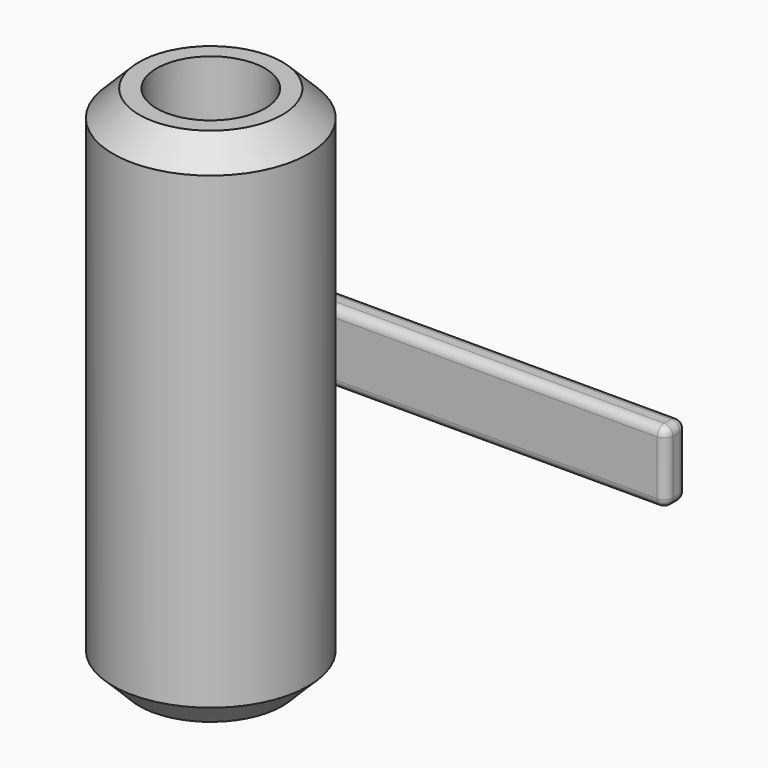
from build123d import *

# Parameters (mm, degrees)
F0_R          = 7.9375
F0_R_2        = 6.35
F2_DEPTH      = 50.8
F3_R          = 14.2875
F3_R_2        = 7.9375
F4_DEPTH      = 63.5
F4_DEPTH_BACK = 12.7
F5_SIZE       = 3.81
F7_START      = -13.97
F6_W          = 64.1522035003
F6_H          = 10.4847997427
F7_DEPTH      = 3.81
F8_T1_DEPTH   = 66.0572035003
F8_T3_DEPTH   = 16.8347997427
F8_T5_DEPTH   = 7.9447997427
F8_T7_DEPTH   = 1.27
F8_S11_W      = 1.27
F8_S11_H      = 1.27
F8_T12_DEPTH  = 1.27
F8_S17_W      = 1.27
F8_S17_H      = 1.27
F8_T18_DEPTH  = 1.27
F8_S23_W      = 1.27
F8_S23_H      = 1.27
F8_T24_DEPTH  = 1.27
F8_S29_W      = 1.27
F8_S29_H      = 1.27
F8_T30_DEPTH  = 1.27
F8_T36_DEPTH  = 54.3607688419
F8_S37_R      = 14.2875
F8_T38_DEPTH  = 29
F8_T42_DEPTH  = 54.3607688419
F8_S43_R      = 14.2875
F8_T44_DEPTH  = 29
F8_T48_DEPTH  = 12.0558566395
F8_S49_R      = 14.2875
F8_T50_DEPTH  = 8
F8_T54_DEPTH  = 12.0558566395
F8_S55_R      = 14.2875
F8_T56_DEPTH  = 8


# Not quite as in the source:
# - a fillet or chamfer that OpenCascade refuses, or shapes differently, is made with other operations: its cross-section is extruded or revolved along the edge and cut away or added
# - a feature names something its author has since deleted; it is built from what else it names


with BuildPart() as f2:
    # F0 (on Top) → F2 (new body)
    with BuildSketch(Plane.XY):
        Circle(F0_R)
        Circle(F0_R_2, mode=Mode.SUBTRACT)
    extrude(amount=F2_DEPTH)

    # F3 (on face) → F4 (join, two sides)
    with BuildSketch(Plane.XY) as f4_sk:
        Circle(F3_R)
        Circle(F3_R_2, mode=Mode.SUBTRACT)
    extrude(amount=F4_DEPTH)
    extrude(f4_sk.sketch, amount=-F4_DEPTH_BACK)

    # F5
    f5_edges = [f2.edges().sort_by_distance(p)[0] for p in [
        (-14.2875, 0, 63.5),
        (-14.2875, 0, -12.7),
    ]]
    chamfer(f5_edges, length=F5_SIZE)

    # F6 (on Front) → F7 (join)
    with BuildSketch(Plane.XZ.offset(F7_START)):
        with Locations((23.3749561012, 26.5372619033)):
            Rectangle(F6_W, F6_H)
    extrude(amount=-F7_DEPTH)

    # F8: fillet of radius 1.27 on 11 edges, made by hand

    # F8_s2 → F8_t1 (cut)
    with BuildSketch(Plane.YZ.offset(-11.876145649)):
        with BuildLine():
            ThreePointArc((16.51, 31.7796617746), (17.4080256121, 31.4076873867), (17.78, 30.5096617746))
            Line((17.78, 30.5096617746), (17.78, 31.7796617746))
            Line((17.78, 31.7796617746), (16.51, 31.7796617746))
        make_face()
        with BuildLine():
            ThreePointArc((16.51, 21.2948620319), (17.4080256121, 21.6668364198), (17.78, 22.5648620319))
            Line((17.78, 22.5648620319), (17.78, 21.2948620319))
            Line((17.78, 21.2948620319), (16.51, 21.2948620319))
        make_face()
    extrude(amount=F8_T1_DEPTH, mode=Mode.SUBTRACT)

    # F8_s4 → F8_t3 (cut)
    with BuildSketch(Plane.XY.offset(18.1198620319)):
        with BuildLine():
            ThreePointArc((-7.431145649, 17.78), (-8.3291712611, 17.4080256121), (-8.701145649, 16.51))
            Line((-8.701145649, 16.51), (-8.701145649, 17.78))
            Line((-8.701145649, 17.78), (-7.431145649, 17.78))
        make_face()
    extrude(amount=F8_T3_DEPTH, mode=Mode.SUBTRACT)

    # F8_s6 → F8_t5 (cut)
    with BuildSketch(Plane.XY.offset(22.5648620319)):
        with BuildLine():
            ThreePointArc((54.1810578513, 13.97), (55.0790834634, 14.3419743879), (55.4510578513, 15.24))
            Line((55.4510578513, 15.24), (55.4510578513, 13.97))
            Line((55.4510578513, 13.97), (54.1810578513, 13.97))
        make_face()
        with BuildLine():
            ThreePointArc((55.4510578513, 16.51), (55.0790834634, 17.4080256121), (54.1810578513, 17.78))
            Line((54.1810578513, 17.78), (55.4510578513, 17.78))
            Line((55.4510578513, 17.78), (55.4510578513, 16.51))
        make_face()
    extrude(amount=F8_T5_DEPTH, mode=Mode.SUBTRACT)

    # F8_s8 → F8_t7 (cut)
    with BuildSketch(Plane.XZ.offset(-16.51)):
        with BuildLine():
            ThreePointArc((54.1810578513, 31.7796617746), (55.0790834634, 31.4076873867), (55.4510578513, 30.5096617746))
            Line((55.4510578513, 30.5096617746), (55.4510578513, 31.7796617746))
            Line((55.4510578513, 31.7796617746), (54.1810578513, 31.7796617746))
        make_face()
        with BuildLine():
            ThreePointArc((54.1810578513, 21.2948620319), (55.0790834634, 21.6668364198), (55.4510578513, 22.5648620319))
            Line((55.4510578513, 22.5648620319), (55.4510578513, 21.2948620319))
            Line((55.4510578513, 21.2948620319), (54.1810578513, 21.2948620319))
        make_face()
    extrude(amount=F8_T7_DEPTH, mode=Mode.SUBTRACT)


with BuildPart() as f8_tool10:
    # F8_s11 → F8_t12 (new body)
    with BuildSketch(Plane.XY.offset(30.5096617746)):
        with Locations((54.8160578513, 17.145)):
            Rectangle(F8_S11_W, F8_S11_H)
    extrude(amount=F8_T12_DEPTH)

    # F8_s13 → F8_t14 (revolve, cut)
    with BuildSketch(Plane(origin=(54.1810578513, 16.51, 30.5096617746), x_dir=(-0.7071067812, -0.7071067812, 0), z_dir=(-0.7071067812, 0.7071067812, 0))):
        with BuildLine():
            ThreePointArc((0, -1.27), (1.27, 0), (0, 1.27))
            Line((0, 1.27), (0, -1.27))
        make_face()
    revolve(axis=Axis((54.1810578513, 16.51, 30.5096617746), (0, 0, 1)), mode=Mode.SUBTRACT)


with BuildPart() as f2_1:
    add(f2.part)

    # F8_t9: cut F8_tool10
    add(f8_tool10.part, mode=Mode.SUBTRACT)


with BuildPart() as f8_tool16:
    # F8_s17 → F8_t18 (new body)
    with BuildSketch(Plane.YZ.offset(54.1810578513)):
        with Locations((17.145, 21.9298620319)):
            Rectangle(F8_S17_W, F8_S17_H)
    extrude(amount=F8_T18_DEPTH)

    # F8_s19 → F8_t20 (revolve, cut)
    with BuildSketch(Plane(origin=(54.1810578513, 16.51, 22.5648620319), x_dir=(0, -0.7071067812, 0.7071067812), z_dir=(0, 0.7071067812, 0.7071067812))):
        with BuildLine():
            ThreePointArc((0, -1.27), (1.27, 0), (0, 1.27))
            Line((0, 1.27), (0, -1.27))
        make_face()
    revolve(axis=Axis((54.1810578513, 16.51, 22.5648620319), (1, 0, 0)), mode=Mode.SUBTRACT)


with BuildPart() as f2_2:
    add(f2_1.part)

    # F8_t15: cut F8_tool16
    add(f8_tool16.part, mode=Mode.SUBTRACT)


with BuildPart() as f8_tool22:
    # F8_s23 → F8_t24 (new body)
    with BuildSketch(Plane.YZ.offset(54.1810578513)):
        with Locations((14.605, 21.9298620319)):
            Rectangle(F8_S23_W, F8_S23_H)
    extrude(amount=F8_T24_DEPTH)

    # F8_s25 → F8_t26 (revolve, cut)
    with BuildSketch(Plane(origin=(54.1810578513, 15.24, 22.5648620319), x_dir=(0, 0.7071067812, 0.7071067812), z_dir=(0, 0.7071067812, -0.7071067812))):
        with BuildLine():
            ThreePointArc((0, -1.27), (1.27, 0), (0, 1.27))
            Line((0, 1.27), (0, -1.27))
        make_face()
    revolve(axis=Axis((54.1810578513, 15.24, 22.5648620319), (1, 0, 0)), mode=Mode.SUBTRACT)


with BuildPart() as f2_3:
    add(f2_2.part)

    # F8_t21: cut F8_tool22
    add(f8_tool22.part, mode=Mode.SUBTRACT)


with BuildPart() as f8_tool28:
    # F8_s29 → F8_t30 (new body)
    with BuildSketch(Plane.XY.offset(30.5096617746)):
        with Locations((54.8160578513, 14.605)):
            Rectangle(F8_S29_W, F8_S29_H)
    extrude(amount=F8_T30_DEPTH)

    # F8_s31 → F8_t32 (revolve, cut)
    with BuildSketch(Plane(origin=(54.1810578513, 15.24, 30.5096617746), x_dir=(-0.7071067812, 0.7071067812, 0), z_dir=(0.7071067812, 0.7071067812, 0))):
        with BuildLine():
            ThreePointArc((0, -1.27), (1.27, 0), (0, 1.27))
            Line((0, 1.27), (0, -1.27))
        make_face()
    revolve(axis=Axis((54.1810578513, 15.24, 30.5096617746), (0, 0, 1)), mode=Mode.SUBTRACT)


with BuildPart() as f2_4:
    add(f2_3.part)

    # F8_t27: cut F8_tool28
    add(f8_tool28.part, mode=Mode.SUBTRACT)


with BuildPart() as f8_tool34:
    # F8_s35 → F8_t36 (new body)
    with BuildSketch(Plane.YZ.offset(-0.1797109906)):
        with BuildLine():
            ThreePointArc((13.97, 22.5648620319), (14.3419743879, 21.6668364198), (15.24, 21.2948620319))
            Line((15.24, 21.2948620319), (13.97, 21.2948620319))
            Line((13.97, 21.2948620319), (13.97, 22.5648620319))
        make_face()
    extrude(amount=F8_T36_DEPTH)

    # F8_s37 → F8_t38 (cut, symmetric)
    with BuildSketch(Plane.XY.offset(21.9)):
        Circle(F8_S37_R)
    extrude(amount=F8_T38_DEPTH, both=True, mode=Mode.SUBTRACT)


with BuildPart() as f2_5:
    add(f2_4.part)

    # F8_t33: cut F8_tool34
    add(f8_tool34.part, mode=Mode.SUBTRACT)


with BuildPart() as f8_tool40:
    # F8_s41 → F8_t42 (new body)
    with BuildSketch(Plane.YZ.offset(54.1810578513)):
        with BuildLine():
            ThreePointArc((13.97, 30.5096617746), (14.3419743879, 31.4076873867), (15.24, 31.7796617746))
            Line((15.24, 31.7796617746), (13.97, 31.7796617746))
            Line((13.97, 31.7796617746), (13.97, 30.5096617746))
        make_face()
    extrude(amount=-F8_T42_DEPTH)

    # F8_s43 → F8_t44 (cut, symmetric)
    with BuildSketch(Plane.XY.offset(31.1)):
        Circle(F8_S43_R)
    extrude(amount=F8_T44_DEPTH, both=True, mode=Mode.SUBTRACT)


with BuildPart() as f2_6:
    add(f2_5.part)

    # F8_t39: cut F8_tool40
    add(f8_tool40.part, mode=Mode.SUBTRACT)


with BuildPart() as f8_tool46:
    # F8_s47 → F8_t48 (new body)
    with BuildSketch(Plane.YZ.offset(-11.876145649)):
        with BuildLine():
            ThreePointArc((15.24, 21.2948620319), (14.3419743879, 21.6668364198), (13.97, 22.5648620319))
            Line((13.97, 22.5648620319), (13.97, 21.2948620319))
            Line((13.97, 21.2948620319), (15.24, 21.2948620319))
        make_face()
    extrude(amount=F8_T48_DEPTH)

    # F8_s49 → F8_t50 (cut, symmetric)
    with BuildSketch(Plane.XY.offset(21.9)):
        Circle(F8_S49_R)
    extrude(amount=F8_T50_DEPTH, both=True, mode=Mode.SUBTRACT)


with BuildPart() as f2_7:
    add(f2_6.part)

    # F8_t45: cut F8_tool46
    add(f8_tool46.part, mode=Mode.SUBTRACT)


with BuildPart() as f8_tool52:
    # F8_s53 → F8_t54 (new body)
    with BuildSketch(Plane.YZ.offset(0.1797109906)):
        with BuildLine():
            ThreePointArc((13.97, 30.5096617746), (14.3419743879, 31.4076873867), (15.24, 31.7796617746))
            Line((15.24, 31.7796617746), (13.97, 31.7796617746))
            Line((13.97, 31.7796617746), (13.97, 30.5096617746))
        make_face()
    extrude(amount=-F8_T54_DEPTH)

    # F8_s55 → F8_t56 (cut, symmetric)
    with BuildSketch(Plane.XY.offset(31.1)):
        Circle(F8_S55_R)
    extrude(amount=F8_T56_DEPTH, both=True, mode=Mode.SUBTRACT)


with BuildPart() as f2_8:
    add(f2_7.part)

    # F8_t51: cut F8_tool52
    add(f8_tool52.part, mode=Mode.SUBTRACT)


solid = f2_8.part
